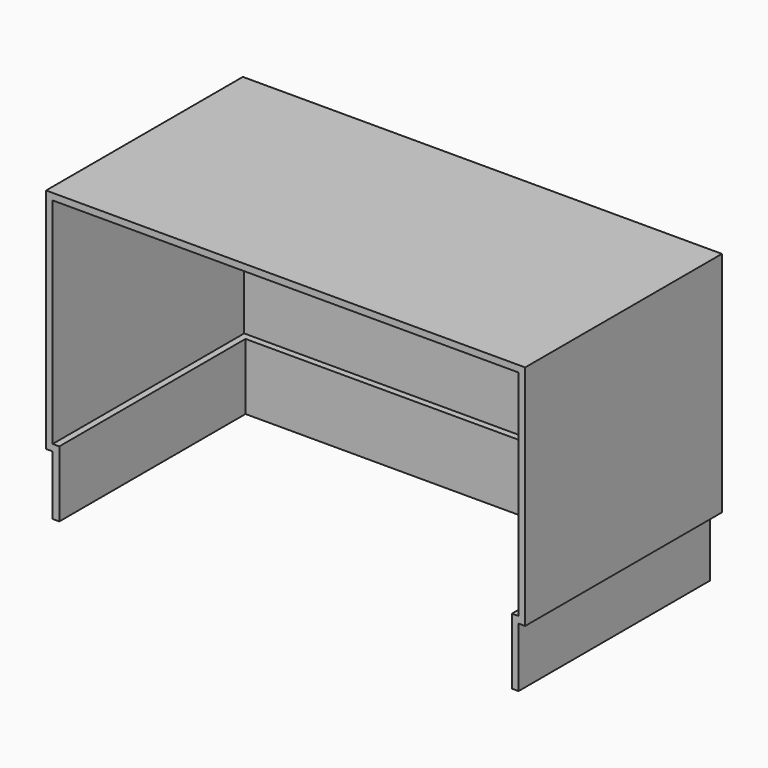
from build123d import *

# Parameters (mm, degrees)
F0_W        = 184.0382497758
F0_H        = 87.4423235655
F1_DEPTH    = 94.488
F2_T        = -2.54
F3_DEPTH    = 25.4
F4_T        = 2.54
F4_T3_DEPTH = 97.028
F4_T5_DEPTH = 184.0382497758
F4_T7_DEPTH = 87.4423235655


# Not quite as in the source:
# - a shell that OpenCascade refuses in one call is made with other operations: the cavity is built on its own and cut out


with BuildPart() as f1:
    # F0 (on Front) → F1 (new body)
    with BuildSketch(Plane.XZ):
        with Locations((72.7289924398, 43.7211617827)):
            Rectangle(F0_W, F0_H)
    extrude(amount=F1_DEPTH)

    # F2
    f2_openings = [f1.faces().sort_by_distance(p)[0] for p in [
        (72.728992, -94.488, 43.721162),
    ]]
    offset(amount=F2_T, openings=f2_openings)

    # F3 (add): a face of the model
    f3_faces = [f1.faces().sort_by_distance(p)[0] for p in [
        (72.7289924398, -48.514, 2.54),
    ]]
    extrude(f3_faces, amount=-F3_DEPTH)

    # F4: shell of thickness 2.54, made by hand


with BuildPart() as f4_core1:
    # F4_t2: copy of F1
    add(f1.part)

    # the walls: a layer under each face that stays
    f4_faces = [f4_core1.faces().sort_by_distance(p)[0] for p in [
        (-19.2901324481, -47.244, 43.7211617827),
        (72.7289924398, -47.244, 87.4423235655),
        (104.36056662, -2.333037037, 0),
        (72.7289924398, 0, 43.7211617827),
        (164.7481173277, -47.244, 43.7211617827),
        (162.2081173277, -48.514, -11.43),
        (72.7289924398, -2.54, -11.43),
        (-16.7501324481, -48.514, -11.43),
        (162.2081173277, -48.514, 43.7211617827),
        (72.7289924398, -48.514, 84.9023235655),
        (-16.7501324481, -48.514, 43.7211617827),
        (72.7289924398, -2.54, 43.7211617827),
    ]]
    thicken(f4_faces, amount=-F4_T, mode=Mode.SUBTRACT)

    # F4_s4 → F4_t3 (cut)
    with BuildSketch(Plane.XZ):
        Polygon((162.2335173277, -0.0254), (162.2081173277, 2.54), (159.6681173277, 2.54), (159.6681173277, 0), align=None)
        Polygon((-16.7755324481, -0.0254), (-16.7501324481, 2.54), (-14.2101324481, 2.54), (-14.2101324481, 0), align=None)
        Polygon((162.1827173277, 84.8769235655), (164.7481173277, 84.9023235655), (164.7481173277, 87.4423235655), (162.2081173277, 87.4423235655), align=None)
        Polygon((-16.7247324481, 84.8769235655), (-16.7501324481, 87.4423235655), (-19.2901324481, 87.4423235655), (-19.2901324481, 84.9023235655), align=None)
    extrude(amount=F4_T3_DEPTH, mode=Mode.SUBTRACT)

    # F4_s6 → F4_t5 (cut)
    with BuildSketch(Plane.YZ.offset(-19.2901324481)):
        Polygon((-2.5146, -0.0254), (-2.54, 2.54), (-5.08, 2.54), (-5.08, 0), align=None)
        Polygon((-2.5654, 84.8769235655), (-2.54, 87.4423235655), (0, 87.4423235655), (0, 84.9023235655), align=None)
    extrude(amount=F4_T5_DEPTH, mode=Mode.SUBTRACT)

    # F4_s8 → F4_t7 (cut)
    with BuildSketch(Plane.XY):
        Polygon((162.1827173277, -2.5654), (164.7481173277, -2.54), (164.7481173277, 0), (162.2081173277, 0), align=None)
        Polygon((-16.7247324481, -2.5654), (-19.2901324481, -2.54), (-19.2901324481, 0), (-16.7501324481, 0), align=None)
    extrude(amount=F4_T7_DEPTH, mode=Mode.SUBTRACT)


with BuildPart() as f1_1:
    add(f1.part)

    # what is left inside the walls is the cavity
    f4_cavity = [f4_core1.part.solids().sort_by_distance(p)[0] for p in [
        (72.728992, -64.685333, 2.5146),
    ]]
    add(f4_cavity, mode=Mode.SUBTRACT)


solid = f1_1.part
